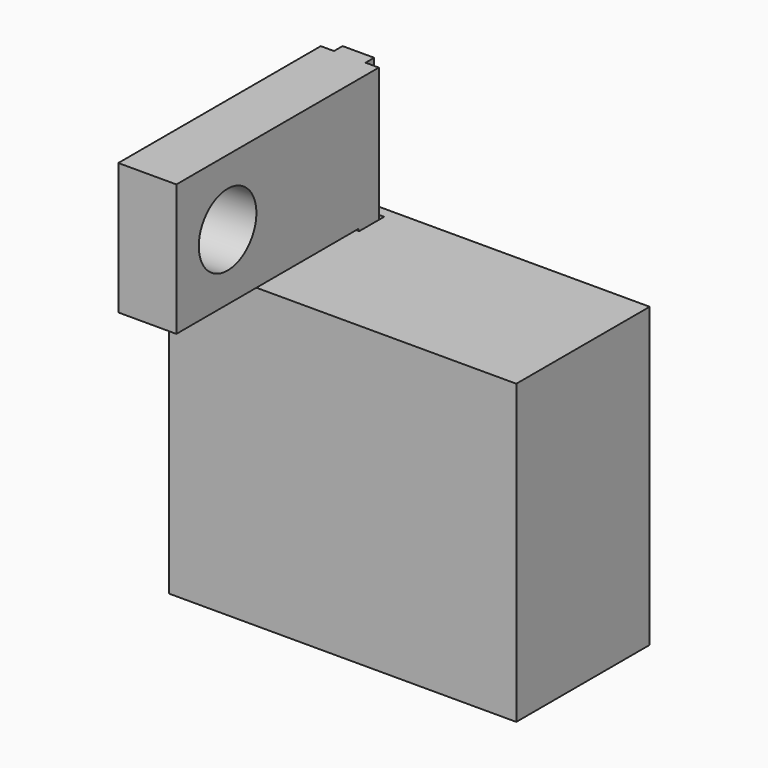
from build123d import *

# Parameters (mm, degrees)
F1_DEPTH = 25.4
F3_DEPTH = 25.4
F5_DEPTH = 11.2268
F6_R     = 3.0734
F7_DEPTH = 4.953


with BuildPart() as f1:
    # F0 (on Top) → F1 (new body)
    with BuildSketch(Plane.XY):
        Polygon((0, -2.667), (0, 0), (1.1303, 0), (1.1303, 0.9144), (-2.2352, 0.9144), (-2.2352, -13.3096), (27.3812, -13.3096), (27.3812, 0.9144), (4.3307, 0.9144), (4.3307, 0), (5.461, 0), (5.461, -2.667), align=None)
    extrude(amount=F1_DEPTH)


with BuildPart() as f3:
    # F2 (on face) → F3 (new body, through all)
    with BuildSketch(Plane.XY.offset(25.4)):
        Polygon((1.3843, -0.254), (0.254, -0.254), (0.254, -2.413), (5.207, -2.413), (5.207, -0.254), (4.0767, -0.254), (4.0767, 0.6604), (1.3843, 0.6604), align=None)
    extrude(amount=-F3_DEPTH)

    # F4 (on face) → F5 (join)
    with BuildSketch(Plane.XY.offset(25.4)):
        Polygon((1.3843, -0.254), (0.254, -0.254), (0.254, -21.844), (5.207, -21.844), (5.207, -0.254), (4.0767, -0.254), (4.0767, 0.6604), (1.3843, 0.6604), align=None)
    extrude(amount=F5_DEPTH)

    # F6 (on face) → F7 (cut, through all)
    with BuildSketch(Plane(origin=(0.254, 0, 0), x_dir=(0, -1, 0), z_dir=(-1, 0, 0))):
        with Locations((16.383, 31.0134)):
            Circle(F6_R)
    extrude(amount=-F7_DEPTH, mode=Mode.SUBTRACT)


solid = Compound([f1.part, f3.part])
